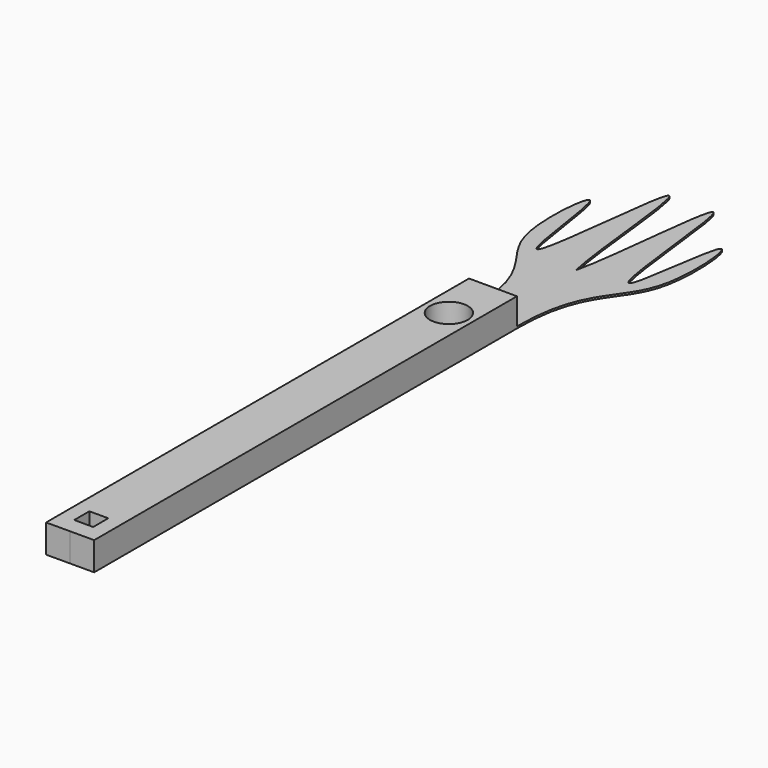
from build123d import *

# Parameters (mm, degrees)
F0_R     = 10
F1_DEPTH = 15
F2_DEPTH = 1


# Not quite as in the source:
# - the program builds the solid bodies; features that only make, move or delete a surface that nothing else refers to are left out


with BuildPart() as f1:
    # F0 (on Top) → F1 (new body)
    with BuildSketch(Plane.XY):
        Polygon((-24.7408044073, 102.8763536353), (-25.3227068062, 102.8771928915), (-25.4, -176.6965887547), (-12.7000101117, -176.6627696025), (0, -176.6376685866), (0.0772667763, 102.8405594523), align=None)
        Polygon((-7.6882185823, -167.7120473838), (-12.6882185823, -167.7120473838), (-17.6882185823, -167.7120473838), (-17.6882185823, -157.7120473838), (-7.6882185823, -157.7120473838), align=None, mode=Mode.SUBTRACT)
        with Locations((-12.5718917698, 73.6229792237)):
            Circle(F0_R, mode=Mode.SUBTRACT)
    extrude(amount=F1_DEPTH)

    # F0 (on Top) → F2 (join)
    with BuildSketch(Plane.XY):
        with BuildLine():
            add(Edge.make_bspline(
                [(-24.7408044073, 102.8763536353), (-24.5499731224, 146.3058625973), (-56.1264111013, 148.8115226622), (-46.337718937, 244.1291976069), (-35.7951301844, 108.7183096569), (-23.6763074235, 294.8900000324), (-17.3487418132, 180.0091377711), (-12.2603111545, 157.1042177733)],
                knots=[5.1182e-06, 5.1182e-06, 5.1182e-06, 5.1182e-06, 0.2151732827, 0.3772222016, 0.5556150865, 0.7731213903, 0.9948403354, 0.9948403354, 0.9948403354, 0.9948403354], degree=3))
            Line((-24.7408044073, 102.8763536353), (0.0772667763, 102.8405594523))
            add(Edge.make_bspline(
                [(0.0772667763, 102.8405594523), (0, 146.2734540246), (31.583875119, 148.6950964448), (22.0462684069, 244.039109704), (11.1469408614, 108.6564689703), (-0.4813218442, 294.8594433526), (-7.1115491577, 179.9956514674), (-12.2603111545, 157.1042177733)],
                knots=[0, 0, 0, 0, 0.2151732827, 0.3772222016, 0.5556150865, 0.7731213903, 0.9948403354, 0.9948403354, 0.9948403354, 0.9948403354], degree=3))
        make_face()
    extrude(amount=F2_DEPTH)


solid = f1.part
